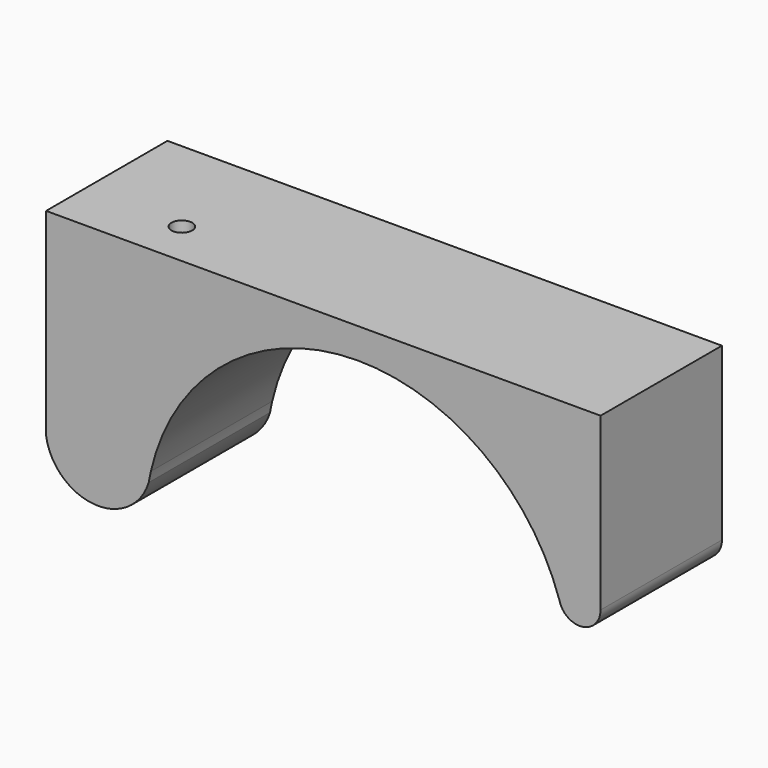
from build123d import *

# Parameters (mm, degrees)
F1_DEPTH = 15.875
F2_R     = 1.0922
F3_DEPTH = 12.7


# Not quite as in the source:
# - ends of sketch curves that miss each other by under 0.0002 mm in the source are joined


with BuildPart() as f1:
    # F0 (on Front) → F1 (new body)
    with BuildSketch(Plane.XZ):
        with BuildLine():
            ThreePointArc((21.0836389118, 7.0307037512), (21.1482213946, 6.8339854292), (21.2109684651, 6.6366739991))
            ThreePointArc((21.2109684651, 6.6366739991), (22.5210215532, 5.4318172042), (24.2927235367, 5.6020848515))
            Line((24.2927235367, 5.6020848515), (24.5564028335, 5.7779212439))
            ThreePointArc((24.5564028335, 5.7779212439), (24.6317726398, 5.83924537), (24.7043401509, 5.9038612541))
            ThreePointArc((24.7043401509, 5.9038612541), (24.1693958795, 7.8102690619), (23.4875772319, 9.6692148479))
            ThreePointArc((23.4875772319, 9.6692148479), (21.6017035502, 8.9730623402), (21.0836389118, 7.0307037512))
        make_face()
        with BuildLine():
            ThreePointArc((-25.3984668781, 0.2790703183), (-23.2092642977, 1.6544209311), (-21.8846396204, 3.8746836882))
            ThreePointArc((-21.8846396204, 3.8746836882), (-21.7800085202, 4.4251388519), (-21.6615343316, 4.9727814551))
            ThreePointArc((-21.6615343316, 4.9727814551), (-21.6412555699, 5.2455472098), (-21.6344904646, 5.5189820621))
            ThreePointArc((-21.6344904646, 5.5189820621), (-22.1206425964, 7.786095443), (-23.4936109358, 9.6545453128))
            ThreePointArc((-23.4936109358, 9.6545453128), (-24.8914383088, 5.057301545), (-25.3984668781, 0.2790703183))
        make_face()
        with BuildLine():
            Line((0, 25.4), (0, 22.225))
            ThreePointArc((0, 22.225), (12.9940993172, 18.0306408077), (21.0836389118, 7.0307037512))
            ThreePointArc((21.0836389118, 7.0307037512), (21.6017035502, 8.9730623402), (23.4875772319, 9.6692148479))
            ThreePointArc((23.4875772319, 9.6692148479), (14.1343896731, 21.1040050362), (0, 25.4))
        make_face()
        with BuildLine():
            ThreePointArc((-21.6615343316, 4.9727814551), (-13.8461286495, 17.3849172106), (0, 22.225))
            Line((0, 22.225), (0, 25.4))
            ThreePointArc((0, 25.4), (-14.1409785562, 21.099590647), (-23.4936109358, 9.6545453128))
            ThreePointArc((-23.4936109358, 9.6545453128), (-22.1206425964, 7.786095443), (-21.6344904646, 5.5189820621))
            ThreePointArc((-21.6344904646, 5.5189820621), (-21.6412555699, 5.2455472098), (-21.6615343316, 4.9727814551))
        make_face()
        with BuildLine():
            ThreePointArc((-26.8263954087, 0), (-26.1032119587, 0.0923630453), (-25.3984668781, 0.2790703183))
            ThreePointArc((-25.3984668781, 0.2790703183), (-24.8914383088, 5.057301545), (-23.4936109358, 9.6545453128))
            ThreePointArc((-23.4936109358, 9.6545453128), (-29.0403261825, 10.7200919312), (-32.6289507574, 6.3585310541))
            Line((-32.6289507574, 6.3585310541), (-32.6289507574, 4.6794330701))
            ThreePointArc((-32.6289507574, 4.6794330701), (-30.8909302127, 1.4347070449), (-27.501154691, 0))
            Line((-27.501154691, 0), (-26.8263954087, 0))
        make_face()
        with BuildLine():
            ThreePointArc((23.4875772319, 9.6692148479), (24.1693958795, 7.8102690619), (24.7043401509, 5.9038612541))
            ThreePointArc((24.7043401509, 5.9038612541), (25.2185681707, 6.630615454), (25.4000290489, 7.5022082908))
            ThreePointArc((25.4000290489, 7.5022082908), (24.8535428533, 8.9473198237), (23.4875772319, 9.6692148479))
        make_face()
        with BuildLine():
            ThreePointArc((23.4875772319, 9.6692148479), (24.8535428533, 8.9473198237), (25.4000290489, 7.5022082908))
            Line((25.4000290489, 7.5022082908), (25.4, 25.4))
            Line((25.4, 25.4), (0, 25.4))
            ThreePointArc((0, 25.4), (14.1343896731, 21.1040050362), (23.4875772319, 9.6692148479))
        make_face()
        with BuildLine():
            ThreePointArc((-23.4936109358, 9.6545453128), (-14.1409785562, 21.099590647), (0, 25.4))
            Line((0, 25.4), (-25.3993433231, 25.4))
            Line((-25.3993433231, 25.4), (-32.6289507574, 25.4))
            Line((-32.6289507574, 25.4), (-32.6289507574, 6.3585310541))
            ThreePointArc((-32.6289507574, 6.3585310541), (-29.0403261825, 10.7200919312), (-23.4936109358, 9.6545453128))
        make_face()
    extrude(amount=F1_DEPTH)

    # F2 (on face) → F3 (cut)
    with BuildSketch(Plane.XY.offset(25.4)):
        with Locations((-22.225, -11.1125)):
            Circle(F2_R)
    extrude(amount=-F3_DEPTH, mode=Mode.SUBTRACT)


solid = f1.part
